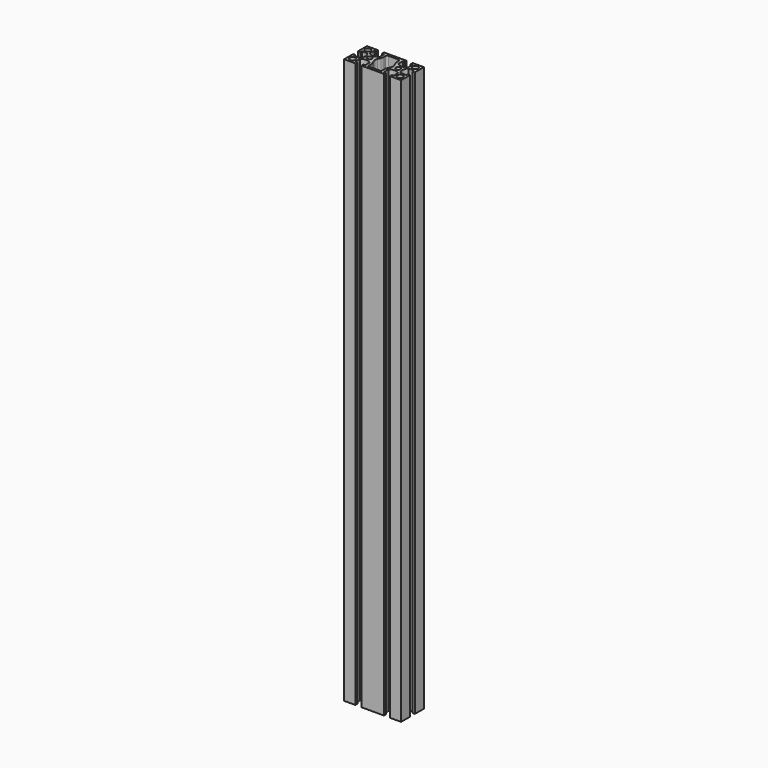
from build123d import *

# Parameters (mm, degrees)
F0_R     = 3
F0_R_2   = 2.5
F1_DEPTH = 595
F2_R     = 2
F3_R     = 7


# Not quite as in the source:
# - a feature names something its author has since deleted; it is built from what else it names


with BuildPart() as f1:
    # F0 (on Top) → F1 (new body)
    with BuildSketch(Plane.XY):
        with BuildLine():
            Line((18.15, -15), (30, -15))
            Line((30, -15), (30, -3.15))
            Line((30, -3.15), (27.5, -3.15))
            Line((27.5, -3.15), (27.5, -5.15))
            Line((27.5, -5.15), (21.5477069044, -5.15))
            ThreePointArc((21.5477069044, -5.15), (19.5, 0), (21.5477069044, 5.15))
            Line((21.5477069044, 5.15), (27.5, 5.15))
            Line((27.5, 5.15), (27.5, 3.15))
            Line((27.5, 3.15), (30, 3.15))
            Line((30, 3.15), (30, 15))
            Line((30, 15), (18.15, 15))
            Line((18.15, 15), (18.15, 12.5))
            Line((18.15, 12.5), (20.15, 12.5))
            Line((20.15, 12.5), (20.15, 6.5477069044))
            ThreePointArc((20.15, 6.5477069044), (15, 4.5), (9.85, 6.5477069044))
            Line((9.85, 6.5477069044), (9.85, 12.5))
            Line((9.85, 12.5), (11.85, 12.5))
            Line((11.85, 12.5), (11.85, 15))
            Line((11.85, 15), (-11.85, 15))
            Line((-11.85, 15), (-11.85, 12.5))
            Line((-11.85, 12.5), (-9.85, 12.5))
            Line((-9.85, 12.5), (-9.85, 6.5477069044))
            ThreePointArc((-9.85, 6.5477069044), (-15, 4.5), (-20.15, 6.5477069044))
            Line((-20.15, 6.5477069044), (-20.15, 12.5))
            Line((-20.15, 12.5), (-18.15, 12.5))
            Line((-18.15, 12.5), (-18.15, 15))
            Line((-18.15, 15), (-30, 15))
            Line((-30, 15), (-30, 3.15))
            Line((-30, 3.15), (-27.5, 3.15))
            Line((-27.5, 3.15), (-27.5, 5.15))
            Line((-27.5, 5.15), (-21.5477069044, 5.15))
            ThreePointArc((-21.5477069044, 5.15), (-19.5, 0), (-21.5477069044, -5.15))
            Line((-21.5477069044, -5.15), (-27.5, -5.15))
            Line((-27.5, -5.15), (-27.5, -3.15))
            Line((-27.5, -3.15), (-30, -3.15))
            Line((-30, -3.15), (-30, -15))
            Line((-30, -15), (-18.15, -15))
            Line((-18.15, -15), (-18.15, -12.5))
            Line((-18.15, -12.5), (-20.15, -12.5))
            Line((-20.15, -12.5), (-20.15, -6.5477069044))
            ThreePointArc((-20.15, -6.5477069044), (-15, -4.5), (-9.85, -6.5477069044))
            Line((-9.85, -6.5477069044), (-9.85, -12.5))
            Line((-9.85, -12.5), (-11.85, -12.5))
            Line((-11.85, -12.5), (-11.85, -15))
            Line((-11.85, -15), (11.85, -15))
            Line((11.85, -15), (11.85, -12.5))
            Line((11.85, -12.5), (9.85, -12.5))
            Line((9.85, -12.5), (9.85, -6.5477069044))
            ThreePointArc((9.85, -6.5477069044), (15, -4.5), (20.15, -6.5477069044))
            Line((20.15, -6.5477069044), (20.15, -12.5))
            Line((20.15, -12.5), (18.15, -12.5))
            Line((18.15, -12.5), (18.15, -15))
        make_face()
        with Locations((-25, -10)):
            Circle(F0_R, mode=Mode.SUBTRACT)
        with Locations((25, -10)):
            Circle(F0_R, mode=Mode.SUBTRACT)
        with Locations((-15, 0)):
            Circle(F0_R_2, mode=Mode.SUBTRACT)
        with Locations((-25, 10)):
            Circle(F0_R, mode=Mode.SUBTRACT)
        Polygon((-7, 7), (-7, 12.5), (0, 12.5), (7, 12.5), (7, 7), (10, 0), (7, -7), (7, -12.5), (0, -12.5), (-7, -12.5), (-7, -7), (-10, 0), align=None, mode=Mode.SUBTRACT)
        with Locations((15, 0)):
            Circle(F0_R_2, mode=Mode.SUBTRACT)
        with Locations((25, 10)):
            Circle(F0_R, mode=Mode.SUBTRACT)
    extrude(amount=F1_DEPTH)

    # F2
    f2_edges = [f1.edges().sort_by_distance(p)[0] for p in [
        (-7, 12.5, 297.5),
        (7, 12.5, 297.5),
    ]]
    fillet(f2_edges, radius=F2_R)

    # F3
    f3_edges = [f1.edges().sort_by_distance(p)[0] for p in [
        (-7, 7, 297.5),
        (-10, 0, 297.5),
        (7, 7, 297.5),
        (10, 0, 297.5),
    ]]
    fillet(f3_edges, radius=F3_R)


solid = f1.part
